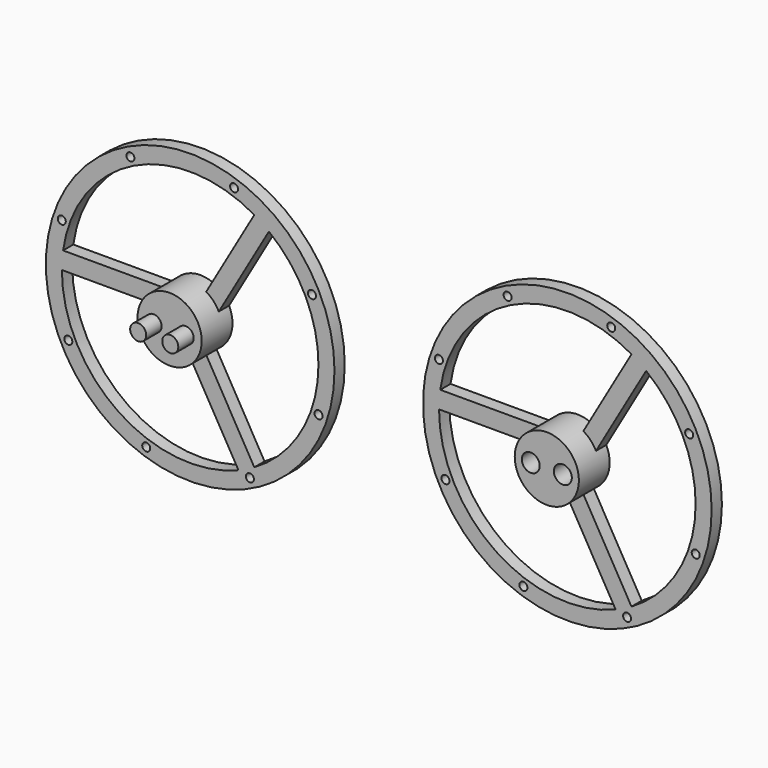
from build123d import *

# Parameters (mm, degrees)
F0_R      = 57.15
F1_DEPTH  = 5.08
F3_DEPTH  = 10.16
F4_R      = 1.5875
F5_DEPTH  = 25.4
F6_R      = 3.175
F8_DEPTH  = 7.62
F11_R     = 2.54
F12_DEPTH = 7.62
F13_W     = 2.159
F13_H     = 5.588
F14_DEPTH = 5.08
F15_R     = 3.556
F15_R_2   = 3.175
F16_DEPTH = 15.24


# Not quite as in the source:
# - a feature names something its author has since deleted; it is built from what else it names


with BuildPart() as f1:
    # F0 (on Front) → F1 (new body)
    with BuildSketch(Plane.XZ):
        Circle(F0_R)
        with BuildLine():
            ThreePointArc((31.1928633958, 40.095452026), (45.6357177028, 22.3163901594), (50.8, 0))
            ThreePointArc((50.8, 0), (43.9940905122, -25.4), (25.4, -43.9940905122))
            Line((25.4, -43.9940905122), (26.8605, -46.5237507167))
            Line((26.8605, -46.5237507167), (20.8276924685, -50.006793769))
            Line((20.8276924685, -50.006793769), (19.1272483329, -47.0615381305))
            ThreePointArc((19.1272483329, -47.0615381305), (-28.3634957709, -42.1444196502), (-50.8, 0))
            Line((-50.8, 0), (-53.721, 0))
            Line((-53.721, 0), (-53.721, 6.9660861045))
            Line((-53.721, 6.9660861045), (-50.3201117287, 6.9660861045))
            ThreePointArc((-50.3201117287, 6.9660861045), (-22.3163901594, 45.6357177028), (25.4, 43.9940905122))
            Line((25.4, 43.9940905122), (26.8605, 46.5237507167))
            Line((26.8605, 46.5237507167), (32.8933075315, 43.0407076644))
            Line((32.8933075315, 43.0407076644), (31.1928633958, 40.095452026))
        make_face(mode=Mode.SUBTRACT)
        with BuildLine():
            Line((11.3423189116, 5.7133004216), (31.1928633958, 40.095452026))
            ThreePointArc((31.1928633958, 40.095452026), (28.3634957709, 42.1444196502), (25.4, 43.9940905122))
            Line((25.4, 43.9940905122), (6.35, 10.9985226281))
            ThreePointArc((6.35, 10.9985226281), (9.2324390364, 8.7207837629), (11.3423189116, 5.7133004216))
        make_face()
        with BuildLine():
            ThreePointArc((19.1272483329, -47.0615381305), (22.3163901594, -45.6357177028), (25.4, -43.9940905122))
            Line((25.4, -43.9940905122), (6.35, -10.9985226281))
            ThreePointArc((6.35, -10.9985226281), (2.9362007614, -12.3559186259), (-0.7232961513, -12.6793865261))
            Line((-0.7232961513, -12.6793865261), (19.1272483329, -47.0615381305))
        make_face()
        with BuildLine():
            Line((-10.6190227603, 6.9660861045), (-50.3201117287, 6.9660861045))
            ThreePointArc((-50.3201117287, 6.9660861045), (-50.6798859303, 3.4912980526), (-50.8, 0))
            Line((-50.8, 0), (-12.7, 0))
            ThreePointArc((-12.7, 0), (-12.1686397978, 3.635134863), (-10.6190227603, 6.9660861045))
        make_face()
        with BuildLine():
            Line((0, 0), (6.35, 10.9985226281))
            ThreePointArc((6.35, 10.9985226281), (-2.9362007614, 12.3559186259), (-10.6190227603, 6.9660861045))
            Line((-10.6190227603, 6.9660861045), (0, 6.9660861045))
            Line((0, 6.9660861045), (0, 0))
        make_face()
        with BuildLine():
            ThreePointArc((12.7, 0), (12.3559186259, 2.9362007614), (11.3423189116, 5.7133004216))
            Line((11.3423189116, 5.7133004216), (6.0328075315, -3.4830430523))
            Line((6.0328075315, -3.4830430523), (0, 0))
            Line((0, 0), (6.35, -10.9985226281))
            ThreePointArc((6.35, -10.9985226281), (10.9985226281, -6.35), (12.7, 0))
        make_face()
        with BuildLine():
            ThreePointArc((-12.7, 0), (-9.2324390364, -8.7207837629), (-0.7232961513, -12.6793865261))
            Line((-0.7232961513, -12.6793865261), (-6.0328075315, -3.4830430523))
            Line((-6.0328075315, -3.4830430523), (0, 0))
            Line((0, 0), (-12.7, 0))
        make_face()
        with BuildLine():
            Line((-12.7, 0), (0, 0))
            Line((0, 0), (0, 6.9660861045))
            Line((0, 6.9660861045), (-10.6190227603, 6.9660861045))
            ThreePointArc((-10.6190227603, 6.9660861045), (-12.1686397978, 3.635134863), (-12.7, 0))
        make_face()
        with BuildLine():
            Line((6.0328075315, -3.4830430523), (11.3423189116, 5.7133004216))
            ThreePointArc((11.3423189116, 5.7133004216), (9.2324390364, 8.7207837629), (6.35, 10.9985226281))
            Line((6.35, 10.9985226281), (0, 0))
            Line((0, 0), (6.0328075315, -3.4830430523))
        make_face()
        with BuildLine():
            ThreePointArc((-0.7232961513, -12.6793865261), (2.9362007614, -12.3559186259), (6.35, -10.9985226281))
            Line((6.35, -10.9985226281), (0, 0))
            Line((0, 0), (-6.0328075315, -3.4830430523))
            Line((-6.0328075315, -3.4830430523), (-0.7232961513, -12.6793865261))
        make_face()
        with BuildLine():
            ThreePointArc((25.4, 43.9940905122), (28.3634957709, 42.1444196502), (31.1928633958, 40.095452026))
            Line((31.1928633958, 40.095452026), (32.8933075315, 43.0407076644))
            Line((32.8933075315, 43.0407076644), (26.8605, 46.5237507167))
            Line((26.8605, 46.5237507167), (25.4, 43.9940905122))
        make_face()
        with BuildLine():
            Line((26.8605, -46.5237507167), (25.4, -43.9940905122))
            ThreePointArc((25.4, -43.9940905122), (22.3163901594, -45.6357177028), (19.1272483329, -47.0615381305))
            Line((19.1272483329, -47.0615381305), (20.8276924685, -50.006793769))
            Line((20.8276924685, -50.006793769), (26.8605, -46.5237507167))
        make_face()
        with BuildLine():
            ThreePointArc((-50.8, 0), (-50.6798859303, 3.4912980526), (-50.3201117287, 6.9660861045))
            Line((-50.3201117287, 6.9660861045), (-53.721, 6.9660861045))
            Line((-53.721, 6.9660861045), (-53.721, 0))
            Line((-53.721, 0), (-50.8, 0))
        make_face()
    extrude(amount=F1_DEPTH)

    # F2 (on face) → F3 (join)
    with BuildSketch(Plane.XZ.offset(5.08)):
        with BuildLine():
            ThreePointArc((6.35, -10.9985226281), (10.9985226281, -6.35), (12.7, 0))
            ThreePointArc((12.7, 0), (12.3559186259, 2.9362007614), (11.3423189116, 5.7133004216))
            ThreePointArc((11.3423189116, 5.7133004216), (9.2324390364, 8.7207837629), (6.35, 10.9985226281))
            ThreePointArc((6.35, 10.9985226281), (-2.9362007614, 12.3559186259), (-10.6190227603, 6.9660861045))
            ThreePointArc((-10.6190227603, 6.9660861045), (-12.1686397978, 3.635134863), (-12.7, 0))
            ThreePointArc((-12.7, 0), (-9.2324390364, -8.7207837629), (-0.7232961513, -12.6793865261))
            ThreePointArc((-0.7232961513, -12.6793865261), (2.9362007614, -12.3559186259), (6.35, -10.9985226281))
        make_face()
    extrude(amount=F3_DEPTH)

    # F4 (on face) → F5 (cut)
    with BuildSketch(Plane(origin=(0, 0, 0), x_dir=(-1, 0, 0), z_dir=(0, 1, 0))):
        with Locations((-23.6520785838, -48.2445955276)):
            Circle(F4_R)
        with Locations((-50.838625809, -17.3895354974)):
            Circle(F4_R)
        with Locations((-48.2445955276, 23.6520785838)):
            Circle(F4_R)
        with Locations((-17.3895354974, 50.838625809)):
            Circle(F4_R)
        with Locations((23.6520785838, 48.2445955276)):
            Circle(F4_R)
        with Locations((50.838625809, 17.3895354974)):
            Circle(F4_R)
        with Locations((48.2445955276, -23.6520785838)):
            Circle(F4_R)
        with Locations((17.3895354974, -50.838625809)):
            Circle(F4_R)
    extrude(amount=-F5_DEPTH, mode=Mode.SUBTRACT)


with BuildPart() as f7_1:
    # F7: copy of F1
    add(f1.part.moved(Location((177.292, 0, 0))))


with BuildPart() as f1_1:
    add(f1.part)

    # F6 (on face) → F8 (join)
    with BuildSketch(Plane.XZ.offset(15.24)):
        with Locations((-6.35, 0)):
            Circle(F6_R)
        with BuildLine():
            ThreePointArc((3.175, 0), (6.35, -3.175), (9.525, 0))
            ThreePointArc((9.525, 0), (6.35, 3.175), (3.175, 0))
        make_face()
    extrude(amount=F8_DEPTH)


with BuildPart() as f10_1:
    # F10: copy of F1
    add(f1_1.part.moved(Location((149.352, 0, 0))))

    # F11 (on face) → F12 (cut)
    with BuildSketch(Plane(origin=(0, 0, 0), x_dir=(-1, 0, 0), z_dir=(0, 1, 0))):
        with Locations((-149.352, 0)):
            Circle(F11_R)
    extrude(amount=-F12_DEPTH, mode=Mode.SUBTRACT)

    # F15 (on face) → F16 (cut)
    with BuildSketch(Plane.XZ.offset(22.86)):
        with Locations((155.702, 0)):
            Circle(F15_R)
        with Locations((155.702, 0)):
            Circle(F15_R_2, mode=Mode.SUBTRACT)
        with Locations((143.002, 0)):
            Circle(F15_R)
        with Locations((155.702, 0)):
            Circle(F15_R_2)
        with Locations((6.35, 0)):
            Circle(F15_R_2)
    extrude(amount=-F16_DEPTH, mode=Mode.SUBTRACT)


with BuildPart() as f1_2:
    add(f1_1.part)

    # F13 (on face) → F14 (cut)
    with BuildSketch(Plane(origin=(0, 0, 0), x_dir=(-1, 0, 0), z_dir=(0, 1, 0))):
        Rectangle(F13_W, F13_H)
    extrude(amount=-F14_DEPTH, mode=Mode.SUBTRACT)


solid = Compound([f10_1.part, f1_2.part])
